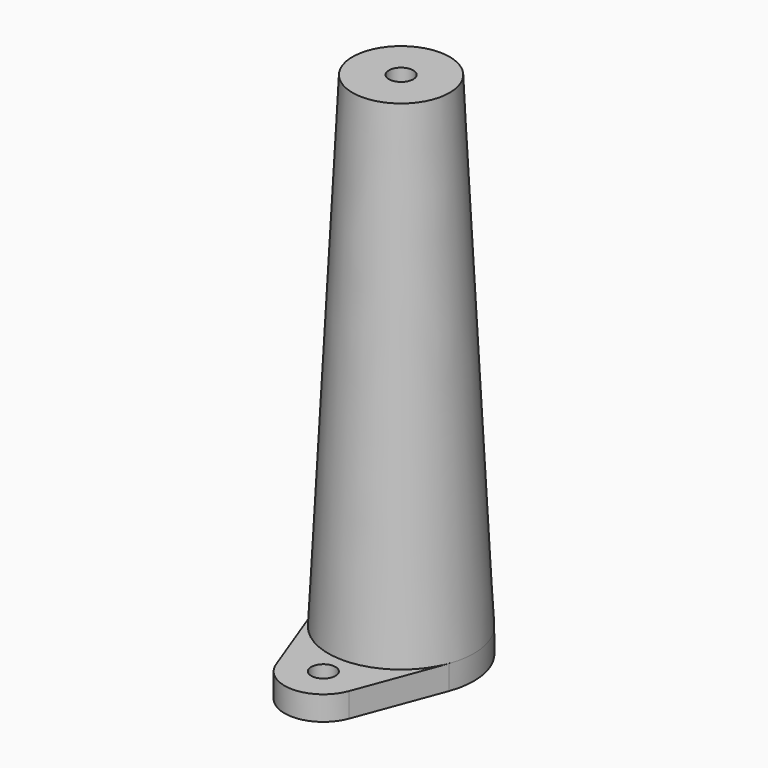
from build123d import *

# Parameters (mm, degrees)
F0_R     = 2.5
F1_DEPTH = 5
F2_R     = 15
F2_R_2   = 2.5
F3_DEPTH = 100
F4_SIZE2 = 99.99999
F4_SIZE  = 4.99999


# Not quite as in the source:
# - a fillet or chamfer is up to 0.001 mm smaller than in the source, because OpenCascade refuses the exact size


with BuildPart() as f1:
    # F0 (on Top) → F1 (new body)
    with BuildSketch(Plane.XY):
        with BuildLine():
            Line((7.4939975981, -22.8), (14.0512454964, -5.25))
            ThreePointArc((14.0512454964, -5.25), (0, 15), (-14.0512454964, -5.25))
            Line((-14.0512454964, -5.25), (-7.4939975981, -22.8))
            ThreePointArc((-7.4939975981, -22.8), (0, -28), (7.4939975981, -22.8))
        make_face()
        with Locations((0, -20)):
            Circle(F0_R, mode=Mode.SUBTRACT)
        Circle(F0_R, mode=Mode.SUBTRACT)
    extrude(amount=F1_DEPTH)

    # F2 (on face) → F3 (join)
    with BuildSketch(Plane.XY.offset(5)):
        Circle(F2_R)
        Circle(F2_R_2, mode=Mode.SUBTRACT)
    extrude(amount=F3_DEPTH)

    # F4 (size 5 and 100 in the source; OpenCascade refuses exactly that, so slightly less here)
    f4_edges = [f1.edges().sort_by_distance(p)[0] for p in [
        (-15, 0, 105),
    ]]
    f4_side = f1.faces().sort_by_distance((-14.575736, 0, 105))[0]
    chamfer(f4_edges, length=F4_SIZE, length2=F4_SIZE2, reference=f4_side)


solid = f1.part
